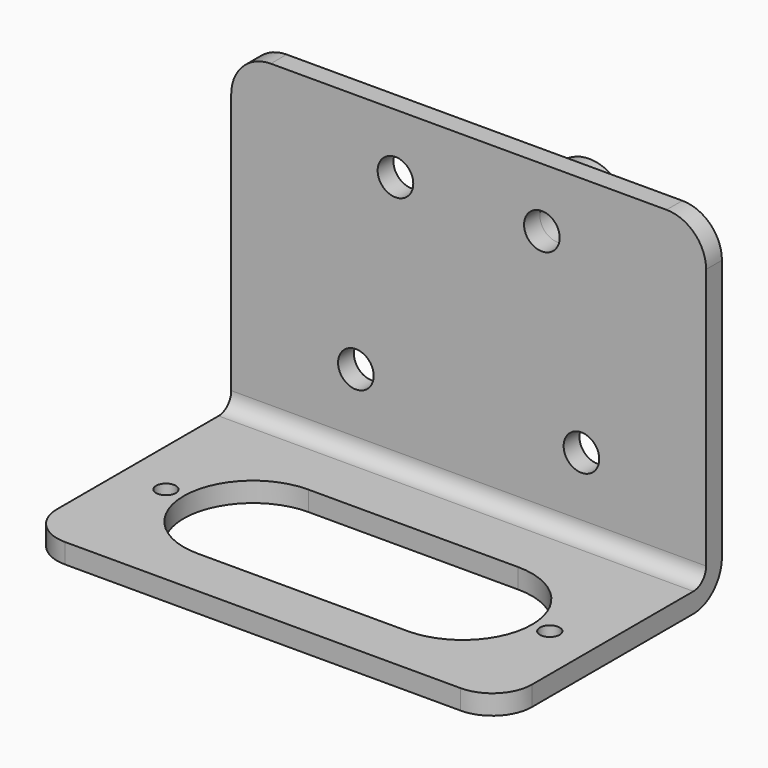
from build123d import *

# Parameters (mm, degrees)
F0_R     = 2.5
F1_DEPTH = 5
F0_R_2   = 4.5
F2_DEPTH = 5
F3_ANGLE = 90
F6_R     = 4
F7_R     = 9
F8_R     = 10
F8_R_2   = 4.5
F9_DEPTH = 10


with BuildPart() as f1:
    # F0 (on Top) → F1 (new body)
    with BuildSketch(Plane.XY):
        with BuildLine():
            Line((60, 0), (-60, 0))
            Line((-60, 0), (-60, -60))
            ThreePointArc((-60, -60), (-57.0710678119, -67.0710678119), (-50, -70))
            Line((-50, -70), (50, -70))
            ThreePointArc((50, -70), (57.0710678119, -67.0710678119), (60, -60))
            Line((60, -60), (60, 0))
        make_face()
        with Locations((-48.5, -40)):
            Circle(F0_R, mode=Mode.SUBTRACT)
        with BuildLine():
            Line((-26.5, -22.5), (26.5, -22.5))
            ThreePointArc((26.5, -22.5), (44, -40), (26.5, -57.5))
            Line((26.5, -57.5), (-26.5, -57.5))
            ThreePointArc((-26.5, -57.5), (-44, -40), (-26.5, -22.5))
        make_face(mode=Mode.SUBTRACT)
        with Locations((48.5, -40)):
            Circle(F0_R, mode=Mode.SUBTRACT)
    extrude(amount=F1_DEPTH)


with BuildPart() as f2:
    # F0 (on Top) → F2 (new body)
    with BuildSketch(Plane.XY):
        with BuildLine():
            Line((-60, 75), (-60, 0))
            Line((-60, 0), (60, 0))
            Line((60, 0), (60, 75))
            ThreePointArc((60, 75), (57.0710678119, 82.0710678119), (50, 85))
            Line((50, 85), (-50, 85))
            ThreePointArc((-50, 85), (-57.0710678119, 82.0710678119), (-60, 75))
        make_face()
        with Locations((-28.5, 24)):
            Circle(F0_R_2, mode=Mode.SUBTRACT)
        with Locations((-18.5, 70)):
            Circle(F0_R_2, mode=Mode.SUBTRACT)
        with Locations((28.5, 24)):
            Circle(F0_R_2, mode=Mode.SUBTRACT)
        with Locations((18.5, 70)):
            Circle(F0_R_2, mode=Mode.SUBTRACT)
    extrude(amount=F2_DEPTH)


with BuildPart() as f2_1:
    # F3: moved
    add(f2.part.rotate(Axis((0, 0, 5), (1, 0, 0)), F3_ANGLE))


with BuildPart() as f2_2:
    # F4: moved
    add(f2_1.part.moved(Location((0, -5, -5))))


with BuildPart() as f1_1:
    add(f1.part)

    # F5: union F2
    add(f2_2.part)

    # F6
    f6_edges = [f1_1.edges().sort_by_distance(p)[0] for p in [
        (0, -5, 5),
    ]]
    fillet(f6_edges, radius=F6_R)

    # F7
    f7_edges = [f1_1.edges().sort_by_distance(p)[0] for p in [
        (0, 0, 0),
    ]]
    fillet(f7_edges, radius=F7_R)


with BuildPart() as f9:
    # F8 (on face) → F9 (new body)
    with BuildSketch(Plane(origin=(0, 0, 0), x_dir=(-1, 0, 0), z_dir=(0, 1, 0))):
        with Locations((-18.5, 70)):
            Circle(F8_R)
        with Locations((-18.5, 70)):
            Circle(F8_R_2, mode=Mode.SUBTRACT)
    extrude(amount=F9_DEPTH)


solid = Compound([f1_1.part, f9.part])
